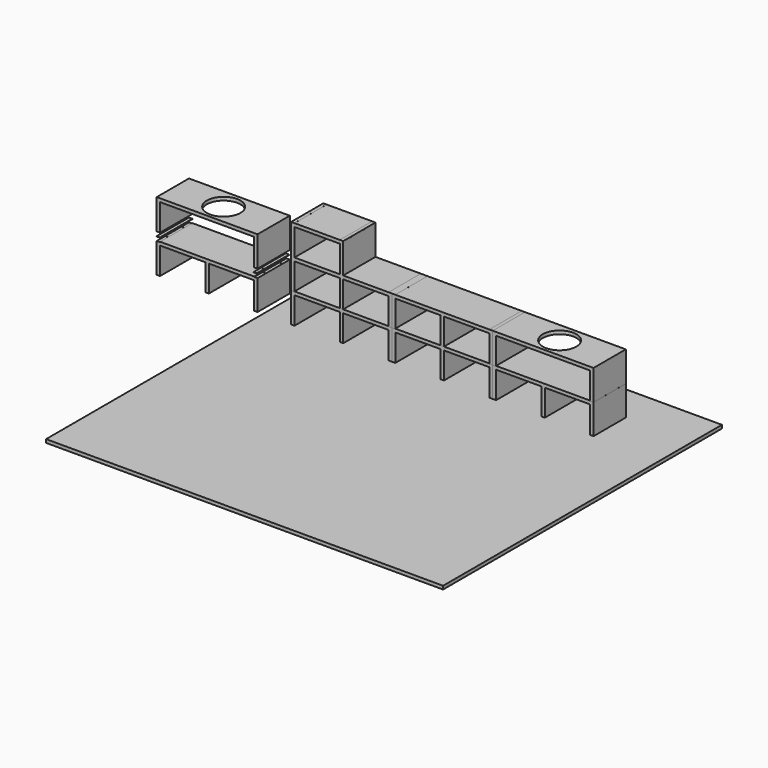
from build123d import *

# Parameters (mm, degrees)
F1_DEPTH  = 609.6
F3_D      = 12.7
F3_DEPTH  = 50.8
F3_TIP    = 3.8154649308
F4_W      = 50.8
F4_H      = 6.35
F5_DEPTH  = 609.6
F7_D      = 6.35
F7_DEPTH  = 6.35
F7_TIP    = 1.9077324654
F9_D      = 6.35
F9_DEPTH  = 6.35
F9_TIP    = 1.9077324654
F11_DEPTH = 609.6
F13_D     = 508
F13_DEPTH = 50.8
F13_TIP   = 152.618597233
F23_W     = 101.346
F23_H     = 6.35
F24_DEPTH = 609.6
F25_W     = 50.8
F25_H     = 6.35
F26_DEPTH = 609.6
F29_W     = 50.8
F29_H     = 609.6
F30_DEPTH = 6.35
F32_DEPTH = 609.6
F33_W     = 50.8
F33_H     = 6.35
F34_DEPTH = 609.6
F38_W     = 6002.2041797638
F38_H     = 5269.7536349297
F39_DEPTH = 50.8


# Not quite as in the source:
# - the program builds the solid bodies; features that only make, move or delete a surface that nothing else refers to are left out


with BuildPart() as f1:
    # F0 (on Front) → F1 (new body)
    with BuildSketch(Plane.XZ):
        Polygon((-110.831476748, 556.6632499456), (-110.831476748, 105.8132499456), (-60.031476748, 105.8132499456), (-60.031476748, 512.2132499456), (625.768523252, 512.2132499456), (625.768523252, 112.1632499456), (676.568523252, 112.1632499456), (676.568523252, 512.2132499456), (1362.368523252, 512.2132499456), (1362.368523252, 105.8132499456), (1413.168523252, 105.8132499456), (1413.168523252, 556.6632499456), (1362.368523252, 556.6632499456), (1362.368523252, 563.0132499456), (-60.031476748, 563.0132499456), (-60.031476748, 556.6632499456), align=None)
    extrude(amount=F1_DEPTH)

    # F3
    with Locations(Plane.XY.offset(556.6632499456)):
        with Locations((-84.6611633897, -146.0916548967), (-84.6611633897, -450.3919780254), (1388.3098363876, -135.5985403061), (1388.3098363876, -450.3919780254)):
            Hole(F3_D / 2, depth=F3_DEPTH)
            with Locations((0, 0, -(F3_DEPTH + F3_TIP / 2))):  # 118° drill point
                Cone(0, F3_D / 2, F3_TIP, mode=Mode.SUBTRACT)


with BuildPart() as f5:
    # F4 (on face) → F5 (new body)
    with BuildSketch(Plane.XZ.offset(609.6)):
        with Locations((-85.431476748, 617.7755988121)):
            Rectangle(F4_W, F4_H)
    extrude(amount=-F5_DEPTH)

    # F7
    with Locations(Plane.XY.offset(620.9505988121)):
        with Locations((-84.4072923064, -137.6516222954), (-84.4072923064, -453.820168972)):
            Hole(F7_D / 2, depth=F7_DEPTH)
            with Locations((0, 0, -(F7_DEPTH + F7_TIP / 2))):  # 118° drill point
                Cone(0, F7_D / 2, F7_TIP, mode=Mode.SUBTRACT)


with BuildPart() as f5b:
    # F4 (on face) → F5, piece 2 (new body)
    with BuildSketch(Plane.XZ.offset(609.6)):
        with Locations((1379.607277298, 617.7755988121)):
            Rectangle(F4_W, F4_H)
    extrude(amount=-F5_DEPTH)

    # F9
    with Locations(Plane.XY.offset(620.9505988121)):
        with Locations((1380.2919387817, -144.1040337086), (1380.2919387817, -466.7250216007)):
            Hole(F9_D / 2, depth=F9_DEPTH)
            with Locations((0, 0, -(F9_DEPTH + F9_TIP / 2))):  # 118° drill point
                Cone(0, F9_D / 2, F9_TIP, mode=Mode.SUBTRACT)


with BuildPart() as f11:
    # F10 (on face) → F11 (new body)
    with BuildSketch(Plane.XZ.offset(609.6)):
        Polygon((-110.831476748, 1141.0505268097), (-110.831476748, 683.8505268097), (-60.031476748, 683.8505268097), (-60.031476748, 1090.2505268097), (1362.368523252, 1090.2505268097), (1362.368523252, 683.8505268097), (1413.168523252, 683.8505268097), (1413.168523252, 1141.0505268097), align=None)
    extrude(amount=-F11_DEPTH)

    # F13
    with Locations(Plane.XY.offset(1141.0505268097)):
        with Locations((660.6196165085, -309.3140423298)):
            Hole(F13_D / 2, depth=F13_DEPTH)
            with Locations((0, 0, -(F13_DEPTH + F13_TIP / 2))):  # 118° drill point
                Cone(0, F13_D / 2, F13_TIP, mode=Mode.SUBTRACT)


with BuildPart() as f14_1:
    # F14: copy of F1
    add(f1.part.moved(Location((2032, 0, 0))))


with BuildPart() as f15_1:
    # F15: copy of F14_1
    add(f14_1.part.moved(Location((0, 0, 450.85))))


with BuildPart() as f16_1:
    # F16: copy of F14_1
    add(f14_1.part.moved(Location((1524, 0, 0))))


with BuildPart() as f17_1:
    # F17: copy of F15_1
    add(f15_1.part.moved(Location((1524, 0, 0))))


with BuildPart() as f18_1:
    # F18: copy of F16_1
    add(f16_1.part.moved(Location((1524, 0, 0))))


with BuildPart() as f19_1:
    # F19: copy of F11
    add(f11.part.moved(Location((5080, 0, -127))))


with BuildPart() as f24:
    # F23 (on face) → F24 (new body)
    with BuildSketch(Plane.XZ.offset(609.6)):
        with Locations((3445.041523252, 1010.6882499456)):
            Rectangle(F23_W, F23_H)
    extrude(amount=-F24_DEPTH)


with BuildPart() as f15_1_1:
    add(f15_1.part)

    # F25 (on face) → F26 (join)
    with BuildSketch(Plane.XZ.offset(609.6)):
        with Locations((1946.568523252, 1010.6882499456)):
            Rectangle(F25_W, F25_H)
    extrude(amount=-F26_DEPTH)

    # F31 (on face) → F32 (join)
    with BuildSketch(Plane.XZ.offset(609.6)):
        Polygon((1921.168523252, 1464.7132499456), (1921.168523252, 1013.8632499456), (1971.968523252, 1013.8632499456), (1971.968523252, 1420.2632499456), (2657.768523252, 1420.2632499456), (2657.768523252, 1013.8632499456), (2708.568523252, 1013.8632499456), (2708.568523252, 1464.7132499456), (2657.768523252, 1464.7132499456), (2657.768523252, 1471.0632499456), (1971.968523252, 1471.0632499456), (1971.968523252, 1464.7132499456), align=None)
    extrude(amount=-F32_DEPTH)


with BuildPart() as f27_1:
    # F27: copy of F11
    add(f11.part.moved(Location((5080, 0, -127))))


with BuildPart() as f30:
    # F29 (on face) → F30 (new body)
    with BuildSketch(Plane.XY.offset(1007.5132499456)):
        with Locations((4943.768523252, -304.8)):
            Rectangle(F29_W, F29_H)
    extrude(amount=F30_DEPTH)


with BuildPart() as f34:
    # F33 (on face) → F34 (new body)
    with BuildSketch(Plane.XZ.offset(609.6)):
        with Locations((1835.7699684143, 1467.8882499456)):
            Rectangle(F33_W, F33_H)
    extrude(amount=-F34_DEPTH)


with BuildPart() as f35_1:
    # F35: copy of F34
    add(f34.part.moved(Location((110.49, 0, 0))))


with BuildPart() as f37_1:
    # F37: copy of F35_1
    add(f35_1.part.moved(Location((736.6, 0, 0))))


with BuildPart() as f39:
    # F38 (on face) → F39 (new body)
    with BuildSketch(Plane(origin=(0, 0, 105.8132499456), x_dir=(1, 0, 0), z_dir=(0, 0, -1))):
        with Locations((4493.7642812729, 2070.0506269932)):
            Rectangle(F38_W, F38_H)
    extrude(amount=F39_DEPTH)


solid = Compound([f1.part, f5.part, f5b.part, f11.part, f14_1.part, f16_1.part, f17_1.part, f18_1.part, f24.part, f15_1_1.part, f27_1.part, f30.part, f35_1.part, f37_1.part, f39.part])
